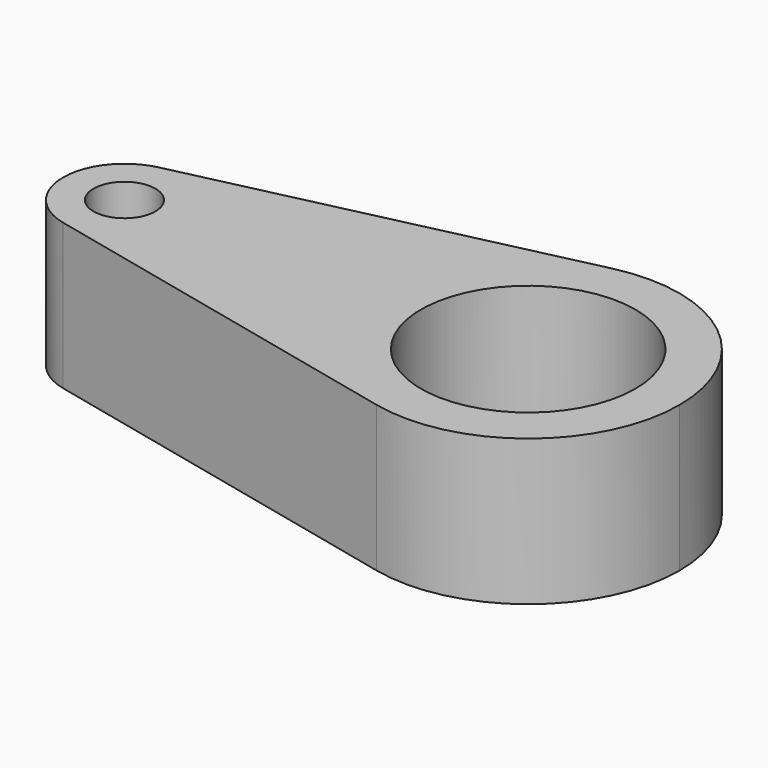
from build123d import *

# Parameters (mm, degrees)
F0_R     = 18.6851980613
F0_R_2   = 5.3827208716
F1_DEPTH = 25.4


# Not quite as in the source:
# - a feature of the source that left no trace in its solid (it failed there, or was rolled back) is left out


with BuildPart() as f1:
    # F0 (on Top) → F1 (new body)
    with BuildSketch(Plane.XY):
        with BuildLine():
            ThreePointArc((-5.8738936456, -25.6938553834), (16.4295502843, -20.6093839908), (26.3567226912, 0))
            ThreePointArc((26.3567226912, 0), (16.4295502843, 20.6093839908), (-5.8738936456, 25.6938553834))
            ThreePointArc((-5.8738936456, 25.6938553834), (-26.3567226912, 0), (-5.8738936456, -25.6938553834))
        make_face()
        Circle(F0_R, mode=Mode.SUBTRACT)
        with BuildLine():
            ThreePointArc((-5.8738936456, -25.6938553834), (-26.3567226912, 0), (-5.8738936456, 25.6938553834))
            Line((-5.8738936456, 25.6938553834), (-72.7058258868, 10.4153517779))
            ThreePointArc((-72.7058258868, 10.4153517779), (-63.6648232454, 8.3542925337), (-59.6407096495, 0))
            ThreePointArc((-59.6407096495, 0), (-63.6648232454, -8.3542925337), (-72.7058258868, -10.4153517779))
            Line((-72.7058258868, -10.4153517779), (-5.8738936456, -25.6938553834))
        make_face()
        with BuildLine():
            ThreePointArc((-59.6407096495, 0), (-63.6648232454, 8.3542925337), (-72.7058258868, 10.4153517779))
            ThreePointArc((-72.7058258868, 10.4153517779), (-81.0088176618, 0), (-72.7058258868, -10.4153517779))
            ThreePointArc((-72.7058258868, -10.4153517779), (-63.6648232454, -8.3542925337), (-59.6407096495, 0))
        make_face()
        with Locations((-70.3247636557, 0)):
            Circle(F0_R_2, mode=Mode.SUBTRACT)
    extrude(amount=F1_DEPTH)


solid = f1.part
